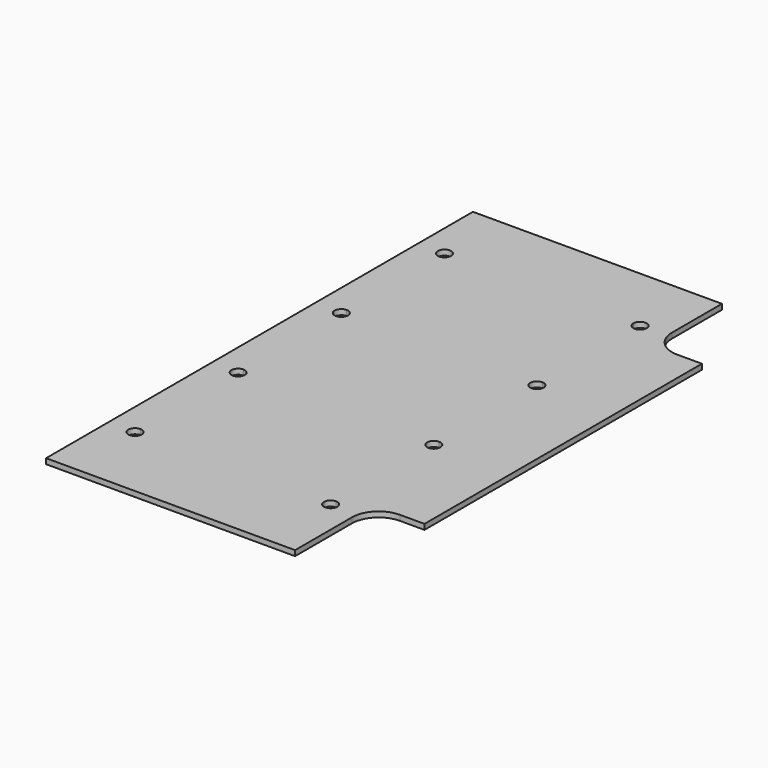
from build123d import *

# Parameters (mm, degrees)
F1_DEPTH = 0.6
F3_DEPTH = 1.201


# Not quite as in the source:
# - a feature names something its author has since deleted; it is built from what else it names


with BuildPart() as f1:
    # F0 (on Top) → F1 (new body, symmetric)
    with BuildSketch(Plane.XY):
        Polygon((56, 120), (0, 120), (0, 106), (0, 0), (56, 0), (56, 16), (56, 106), align=None)
        with BuildLine():
            ThreePointArc((62, 100), (57.7573593129, 101.7573593129), (56, 106))
            Line((56, 106), (56, 16))
            ThreePointArc((56, 16), (57.7573593129, 20.2426406871), (62, 22))
            Line((62, 22), (67.5, 22))
            Line((67.5, 22), (67.5, 100))
            Line((67.5, 100), (62, 100))
        make_face()
    extrude(amount=F1_DEPTH, both=True)

    # F2 (on face) → F3 (cut, through all)
    with BuildSketch(Plane.XY.offset(0.6)):
        with BuildLine():
            Line((6, 103), (6, 104.5))
            Line((6, 104.5), (7.5, 104.5))
            ThreePointArc((7.5, 104.5), (4.9393398282, 105.5606601718), (6, 103))
        make_face()
        with BuildLine():
            Line((7.5, 104.5), (6, 104.5))
            Line((6, 104.5), (6, 103))
            ThreePointArc((6, 103), (7.0606601718, 103.4393398282), (7.5, 104.5))
        make_face()
        with BuildLine():
            ThreePointArc((51.5, 104.5), (50, 106), (48.5, 104.5))
            Line((48.5, 104.5), (50, 104.5))
            Line((50, 104.5), (50, 103))
            ThreePointArc((50, 103), (51.0606601718, 103.4393398282), (51.5, 104.5))
        make_face()
        with BuildLine():
            Line((50, 104.5), (48.5, 104.5))
            ThreePointArc((48.5, 104.5), (48.9393398282, 103.4393398282), (50, 103))
            Line((50, 103), (50, 104.5))
        make_face()
        with BuildLine():
            ThreePointArc((51.5, 75.5), (51.0606601718, 76.5606601718), (50, 77))
            Line((50, 77), (50, 75.5))
            Line((50, 75.5), (50, 74))
            ThreePointArc((50, 74), (51.0606601718, 74.4393398282), (51.5, 75.5))
        make_face()
        with BuildLine():
            Line((50, 75.5), (50, 77))
            ThreePointArc((50, 77), (48.5, 75.5), (50, 74))
            Line((50, 74), (50, 75.5))
        make_face()
        with BuildLine():
            ThreePointArc((51.5, 46.5), (51.0606601718, 47.5606601718), (50, 48))
            Line((50, 48), (50, 46.5))
            Line((50, 46.5), (50, 45))
            ThreePointArc((50, 45), (51.0606601718, 45.4393398282), (51.5, 46.5))
        make_face()
        with BuildLine():
            Line((50, 46.5), (50, 48))
            ThreePointArc((50, 48), (48.5, 46.5), (50, 45))
            Line((50, 45), (50, 46.5))
        make_face()
        with BuildLine():
            ThreePointArc((51.5, 17.5), (51.0606601718, 18.5606601718), (50, 19))
            Line((50, 19), (50, 17.5))
            Line((50, 17.5), (48.5, 17.5))
            ThreePointArc((48.5, 17.5), (50, 16), (51.5, 17.5))
        make_face()
        with BuildLine():
            Line((50, 17.5), (50, 19))
            ThreePointArc((50, 19), (48.9393398282, 18.5606601718), (48.5, 17.5))
            Line((48.5, 17.5), (50, 17.5))
        make_face()
        with BuildLine():
            Line((6, 17.5), (6, 19))
            ThreePointArc((6, 19), (4.9393398282, 16.4393398282), (7.5, 17.5))
            Line((7.5, 17.5), (6, 17.5))
        make_face()
        with BuildLine():
            ThreePointArc((7.5, 17.5), (7.0606601718, 18.5606601718), (6, 19))
            Line((6, 19), (6, 17.5))
            Line((6, 17.5), (7.5, 17.5))
        make_face()
        with BuildLine():
            Line((6, 46.5), (6, 48))
            ThreePointArc((6, 48), (4.5, 46.5), (6, 45))
            Line((6, 45), (6, 46.5))
        make_face()
        with BuildLine():
            ThreePointArc((7.5, 46.5), (7.0606601718, 47.5606601718), (6, 48))
            Line((6, 48), (6, 46.5))
            Line((6, 46.5), (6, 45))
            ThreePointArc((6, 45), (7.0606601718, 45.4393398282), (7.5, 46.5))
        make_face()
        with BuildLine():
            Line((6, 75.5), (6, 77))
            ThreePointArc((6, 77), (4.5, 75.5), (6, 74))
            Line((6, 74), (6, 75.5))
        make_face()
        with BuildLine():
            ThreePointArc((7.5, 75.5), (7.0606601718, 76.5606601718), (6, 77))
            Line((6, 77), (6, 75.5))
            Line((6, 75.5), (6, 74))
            ThreePointArc((6, 74), (7.0606601718, 74.4393398282), (7.5, 75.5))
        make_face()
    extrude(amount=-F3_DEPTH, mode=Mode.SUBTRACT)


solid = f1.part
